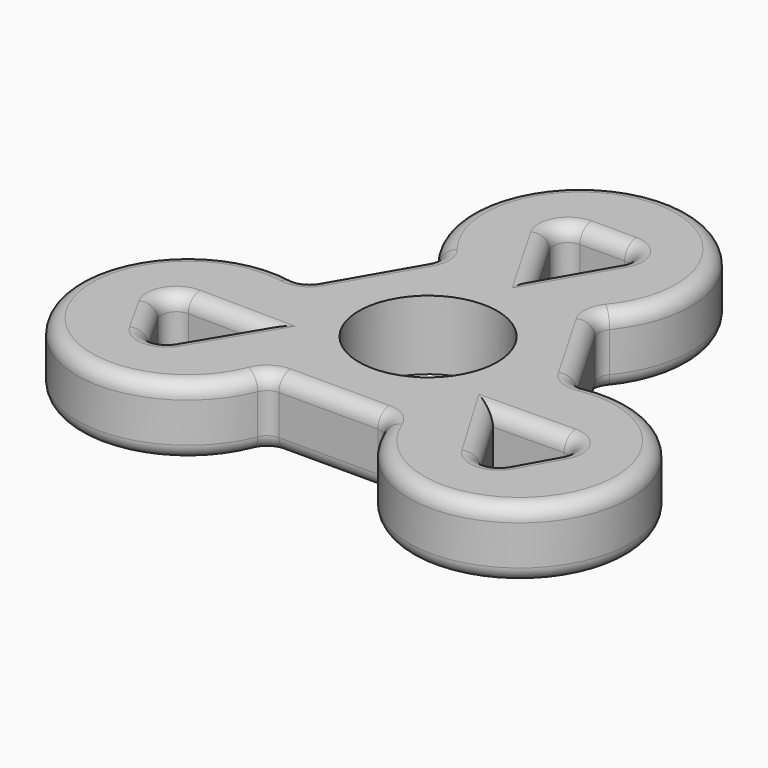
from build123d import *

# Parameters (mm, degrees)
F1_DEPTH = 4.7625
F2_F1_R  = 2.032
F2_F2_R  = 2.032


with BuildPart() as f1:
    # F0 (on Top) → F1 (new body, symmetric)
    with BuildSketch(Plane.XY):
        with BuildLine():
            Line((18.7077457017, 1.8872339495), (10.8635980467, 15.47369623))
            ThreePointArc((10.8635980467, 15.47369623), (0, 41.402), (-10.8635980467, 15.47369623))
            Line((-10.8635980467, 15.47369623), (-18.6962956709, 1.9070659847))
            ThreePointArc((-18.6962956709, 1.9070659847), (-36.2227009747, -20.0746997122), (-8.2621973021, -17.145))
            Line((-8.2621973021, -17.145), (8.2357664047, -17.145))
            ThreePointArc((8.2357664047, -17.145), (36.1902781622, -20.1291440989), (18.7077457017, 1.8872339495))
        make_face()
        Polygon((-29.3987297089, -8.8482320732), (-16.201911861, -9.0411016919), (-22.9673507744, -20.3734463879), align=None, mode=Mode.SUBTRACT)
        Polygon((22.9396512431, -20.4017350098), (16.1886586268, -9.0607783176), (29.3857115337, -8.8847255573), align=None, mode=Mode.SUBTRACT)
        with BuildLine():
            ThreePointArc((0, 9.525), (6.7351920908, 6.7351920908), (9.525, 0))
            ThreePointArc((9.525, 0), (-6.7351920908, -6.7351920908), (0, 9.525))
        make_face(mode=Mode.SUBTRACT)
        Polygon((6.5991135768, 29.972), (0, 18.542), (-6.5991135768, 29.972), align=None, mode=Mode.SUBTRACT)
    extrude(amount=F1_DEPTH, both=True)

    # F2: fillet of radius 2.032 on 24 edges, made by hand

    # F2_f1
    f2_f1_edges = [f1.edges().sort_by_distance(p)[0] for p in [
        (10.8635980467, 15.47369623, 0),
        (-10.8635980467, 15.47369623, 0),
        (-18.6962956709, 1.9070659847, 0),
        (-8.2621973021, -17.145, 0),
        (18.7077457017, 1.8872339495, 0),
        (8.2357664047, -17.145, 0),
        (-29.3987297089, -8.8482320732, 0),
        (-22.9673507744, -20.3734463879, 0),
        (-6.5991135768, 29.972, 0),
        (6.5991135768, 29.972, 0),
        (29.3857115337, -8.8847255573, 0),
        (22.9396512431, -20.4017350098, 0),
    ]]
    fillet(f2_f1_edges, radius=F2_F1_R)

    # F2_f2
    f2_f2_edges = [f1.edges().sort_by_distance(p)[0] for p in [
        (0, 41.402, -4.7625),
        (0, 41.402, 4.7625),
        (-36.2076281274, -20.1021548654, -4.7625),
        (-36.2076281274, -20.1021548654, 4.7625),
        (36.1764741613, -20.1541764802, -4.7625),
        (36.1764741613, -20.1541764802, 4.7625),
        (-26.1830402417, -14.6108392305, -4.7625),
        (-26.1830402417, -14.6108392305, 4.7625),
        (0, 29.972, 4.7625),
        (0, 29.972, -4.7625),
        (26.1626813884, -14.6432302836, -4.7625),
        (26.1626813884, -14.6432302836, 4.7625),
        (27.6396570272, -9.9241088651, 4.7625),
        (22.9125461475, -18.369915797, 4.7625),
        (27.6396570272, -9.9241088651, -4.7625),
        (22.9125461475, -18.369915797, -4.7625),
        (-4.8393499563, 28.956, -4.7625),
        (4.8393499563, 28.956, -4.7625),
        (-4.8393499563, 28.956, 4.7625),
        (4.8393499563, 28.956, 4.7625),
        (-22.9376565541, -18.3416633647, 4.7625),
        (-27.654001106, -9.8898395339, 4.7625),
        (-22.9376565541, -18.3416633647, -4.7625),
        (-27.654001106, -9.8898395339, -4.7625),
        (7.9335935166, -17.4950804933, 4.7625),
        (18.8637972742, 2.3603563212, 4.7625),
        (7.9335935166, -17.4950804933, -4.7625),
        (18.8637972742, 2.3603563212, -4.7625),
        (-18.8525242851, 2.3820174573, 4.7625),
        (-7.9613562378, -17.4940804155, 4.7625),
        (-18.8525242851, 2.3820174573, -4.7625),
        (-7.9613562378, -17.4940804155, -4.7625),
        (11.3342608816, 15.3799323911, 4.7625),
        (-11.3342608816, 15.3799323911, 4.7625),
        (11.3342608816, 15.3799323911, -4.7625),
        (-11.3342608816, 15.3799323911, -4.7625),
    ]]
    fillet(f2_f2_edges, radius=F2_F2_R)


solid = f1.part
